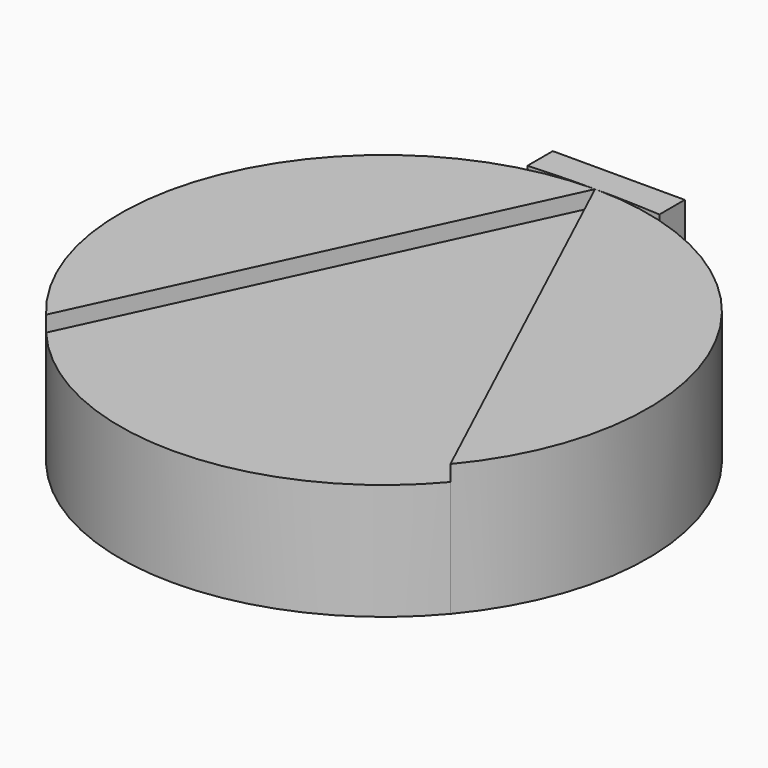
from build123d import *

# Parameters (mm, degrees)
F1_DEPTH = 25
F2_DEPTH = 22


with BuildPart() as f1:
    # F0 (on Top) → F1 (new body)
    with BuildSketch(Plane.XY):
        with BuildLine():
            Line((-38.3022221559, -32.1393804843), (0, 50))
            ThreePointArc((0, 50), (-45.3153893518, 21.130913087), (-38.3022221559, -32.1393804843))
        make_face()
    extrude(amount=F1_DEPTH)


with BuildPart() as f1b:
    # F0 (on Top) → F1, piece 2 (new body)
    with BuildSketch(Plane.XY):
        with BuildLine():
            ThreePointArc((38.3022221559, -32.1393804843), (46.9846310393, -17.1010071663), (50, 0))
            ThreePointArc((50, 0), (35.3553390593, 35.3553390593), (0, 50))
            Line((0, 50), (38.3022221559, -32.1393804843))
        make_face()
    extrude(amount=F1_DEPTH)

    # F0 (on Top) → F2 (join)
    with BuildSketch(Plane.XY):
        with BuildLine():
            Line((38.3022221559, -32.1393804843), (0, 50))
            Line((0, 50), (-38.3022221559, -32.1393804843))
            ThreePointArc((-38.3022221559, -32.1393804843), (0, -50), (38.3022221559, -32.1393804843))
        make_face()
    extrude(amount=F2_DEPTH)


with BuildPart() as f1c:
    # F0 (on Top) → F1, piece 3 (new body)
    with BuildSketch(Plane.XY):
        with BuildLine():
            ThreePointArc((-12.5, 49.6089927834), (-6.2530569853, 49.9022242956), (0, 50))
            ThreePointArc((0, 50), (6.2530569853, 49.9022242956), (12.5, 49.6089927834))
            Line((12.5, 49.6089927834), (12.5, 55.6089927834))
            Line((12.5, 55.6089927834), (-12.5, 55.6089927834))
            Line((-12.5, 55.6089927834), (-12.5, 49.6089927834))
        make_face()
    extrude(amount=F1_DEPTH)


solid = Compound([f1.part, f1b.part, f1c.part])
